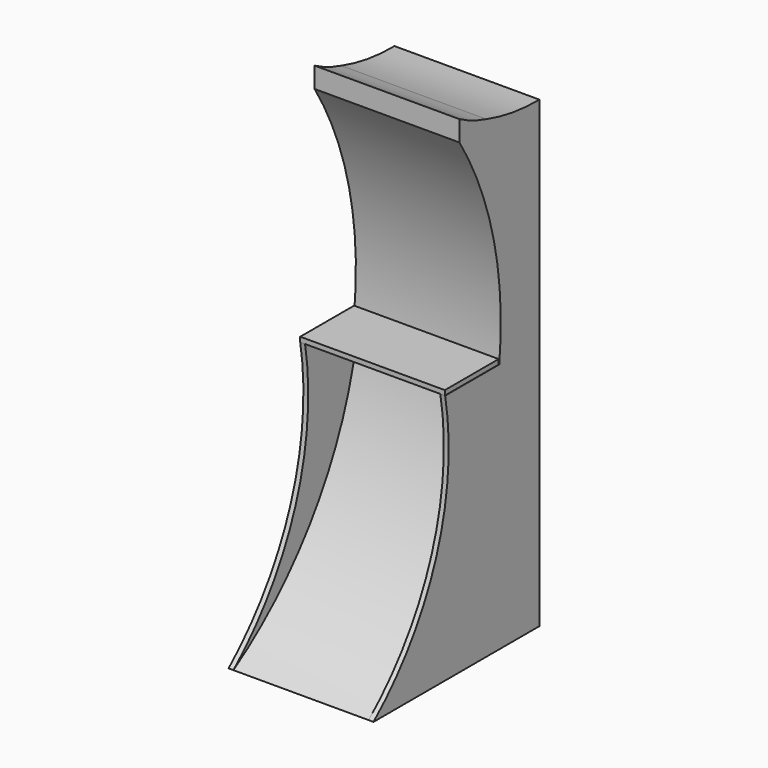
from build123d import *

# Parameters (mm, degrees)
F1_DEPTH  = 600
F3_DEPTH  = 600.001
F5_DEPTH  = 20
F7_DEPTH  = 20
F8_W      = 20
F8_H      = 278.7190201738
F8_W_2    = 578.8190174103
F9_DEPTH  = 20
F10_W     = 598.5316634178
F10_H     = 254.7840774059
F11_DEPTH = 2017.6951884178


# Not quite as in the source:
# - a feature names something its author has since deleted; it is built from what else it names


with BuildPart() as f1:
    # F0 (on Right) → F1 (new body)
    with BuildSketch(Plane.YZ):
        with BuildLine():
            ThreePointArc((-413.7737442203, 1932.6941884178), (-235.6171133469, 874.7152717166), (-858.6646769196, 1.2904570733))
            Line((-858.6646769196, 1.2904570733), (841.3353230804, 1.2904570733))
            ThreePointArc((841.3353230804, 1.2904570733), (218.2877610308, 874.7152723164), (396.4443930804, 1932.6941884178))
            Line((396.4443930804, 1932.6941884178), (396.4443930804, 2017.6941884178))
            ThreePointArc((396.4443930804, 2017.6941884178), (199.7456261802, 1948.7680536266), (-8.6646769196, 1951.2904570733))
            ThreePointArc((-8.6646769196, 1951.2904570733), (-217.0749786293, 1948.7680541113), (-413.7737442203, 2017.6941884178))
            Line((-413.7737442203, 2017.6941884178), (-413.7737442203, 1932.6941884178))
        make_face()
    extrude(amount=F1_DEPTH)

    # F2 (on face) → F3 (cut, through all)
    with BuildSketch(Plane.YZ.offset(600)):
        with BuildLine():
            Line((396.4443930804, 2017.6941884178), (-413.7737442203, 2017.6941884178))
            ThreePointArc((-413.7737442203, 2017.6941884178), (-345.7057427079, 1986.5957603046), (-275.2746839195, 1961.3008790249))
            ThreePointArc((-275.2746839195, 1961.3008790249), (-142.5331399832, 1941.2889121961), (-8.6646769196, 1951.2904570733))
            ThreePointArc((-8.6646769196, 1951.2904570733), (125.2037851776, 1941.2889117025), (257.9453283126, 1961.3008776288))
            ThreePointArc((257.9453283126, 1961.3008776288), (328.3763894007, 1986.5957594221), (396.4443930804, 2017.6941884178))
        make_face()
        with BuildLine():
            ThreePointArc((-8.6646769196, 1951.2904570733), (-142.5331399832, 1941.2889121961), (-275.2746839195, 1961.3008790249))
            ThreePointArc((-275.2746839195, 1961.3008790249), (-8.66467791, 1920.6086514411), (257.9453283126, 1961.3008776288))
            ThreePointArc((257.9453283126, 1961.3008776288), (125.2037851776, 1941.2889117025), (-8.6646769196, 1951.2904570733))
        make_face()
    extrude(amount=-F3_DEPTH, mode=Mode.SUBTRACT)

    # F4 (on face) → F5 (join)
    with BuildSketch(Plane.YZ.offset(600)):
        with BuildLine():
            ThreePointArc((-487.8719790556, 1039.6971702576), (-533.5033840935, 470.5867589871), (-858.6646769196, 1.2904570733))
            ThreePointArc((-858.6646769196, 1.2904570733), (-413.6127871917, 445.5030116798), (-207.8719790556, 1039.6971702576))
            Line((-207.8719790556, 1039.6971702576), (-487.8719790556, 1039.6971702576))
        make_face()
        with BuildLine():
            ThreePointArc((190.5426270267, 1039.6971702576), (396.283434362, 445.5030119538), (841.3353230804, 1.2904570733))
            ThreePointArc((841.3353230804, 1.2904570733), (516.1740306428, 470.5867590462), (470.5426270267, 1039.6971702576))
            Line((470.5426270267, 1039.6971702576), (190.5426270267, 1039.6971702576))
        make_face()
    extrude(amount=-F5_DEPTH)

    # F6 (on face) → F7 (join)
    with BuildSketch(Plane(origin=(0, 0, 0), x_dir=(0, -1, 0), z_dir=(-1, 0, 0))):
        with BuildLine():
            ThreePointArc((-841.3353230804, 1.2904570733), (-396.5475396439, 445.0817710452), (-190.6490020093, 1038.7085012816))
            Line((-190.6490020093, 1038.7085012816), (-470.6490020093, 1038.7085012816))
            ThreePointArc((-470.6490020093, 1038.7085012816), (-519.6815928842, 471.2934981386), (-841.3353230804, 1.2904570733))
        make_face()
        with BuildLine():
            ThreePointArc((207.878498719, 1039.6363848164), (413.6290200403, 445.4771111279), (858.6646769196, 1.2904570733))
            ThreePointArc((858.6646769196, 1.2904570733), (536.7100272294, 471.698228356), (487.878498719, 1039.6363848164))
            Line((487.878498719, 1039.6363848164), (207.878498719, 1039.6363848164))
        make_face()
    extrude(amount=-F7_DEPTH)

    # F8 (on face) → F9 (join)
    with BuildSketch(Plane.XY.offset(1039.6363848164)):
        with Locations((10, -348.5189886321)):
            Rectangle(F8_W, F8_H)
        with Locations((309.4095087051, -348.5189886321)):
            Rectangle(F8_W_2, F8_H)
    extrude(amount=F9_DEPTH)

    # F10 (on Top) → F11 (cut, through all)
    with BuildSketch(Plane.XY):
        Polygon((0, 963.8522267342), (0, 254.7840774059), (598.5316634178, 254.7840774059), (598.5316634178, 0), (664.8825407028, 0), (664.8825407028, 963.8522267342), align=None)
        Polygon((-87.8282785416, 0), (0, 0), (0, 254.7840774059), (0, 963.8522267342), (-87.8282785416, 963.8522267342), align=None)
        with Locations((299.2658317089, 127.392038703)):
            Rectangle(F10_W, F10_H)
    extrude(amount=F11_DEPTH, mode=Mode.SUBTRACT)


solid = f1.part
